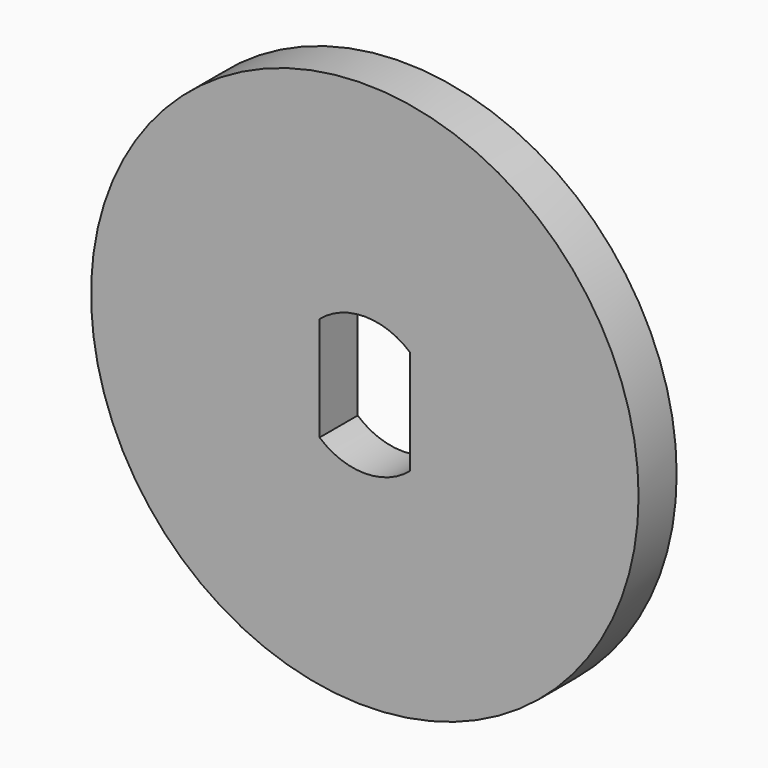
from build123d import *

# Parameters (mm, degrees)
F1_DEPTH = 2
F0_R     = 11.5
F2_DEPTH = 2


# Not quite as in the source:
# - a feature names something its author has since deleted; it is built from what else it names


with BuildPart() as f1:
    # F0 (on Front) → F1 (new body)
    with BuildSketch(Plane.XZ):
        with BuildLine():
            Line((-1.9, -2.19089023), (-1.9, 2.19089023))
            ThreePointArc((-1.9, 2.19089023), (-2.9, 0), (-1.9, -2.19089023))
        make_face()
    extrude(amount=F1_DEPTH)



with BuildPart() as f1b:
    # F0 (on Front) → F1, piece 2 (new body)
    with BuildSketch(Plane.XZ):
        with BuildLine():
            ThreePointArc((1.9, -2.19089023), (2.6381811917, -1.2041594579), (2.9, 0))
            ThreePointArc((2.9, 0), (2.6381811917, 1.2041594579), (1.9, 2.19089023))
            Line((1.9, 2.19089023), (1.9, -2.19089023))
        make_face()
    extrude(amount=F1_DEPTH)


with BuildPart() as f1_1:
    add(f1.part)

    add(f1b.part)  # F2 merges F1b
    # F0 (on Front) → F2 (join)
    with BuildSketch(Plane.XZ):
        Circle(F0_R)
        with BuildLine():
            ThreePointArc((1.9, 2.19089023), (2.6381811917, 1.2041594579), (2.9, 0))
            ThreePointArc((2.9, 0), (2.6381811917, -1.2041594579), (1.9, -2.19089023))
            ThreePointArc((1.9, -2.19089023), (0, -2.9), (-1.9, -2.19089023))
            ThreePointArc((-1.9, -2.19089023), (-2.9, 0), (-1.9, 2.19089023))
            ThreePointArc((-1.9, 2.19089023), (0, 2.9), (1.9, 2.19089023))
        make_face(mode=Mode.SUBTRACT)
    extrude(amount=F2_DEPTH)


solid = f1_1.part
